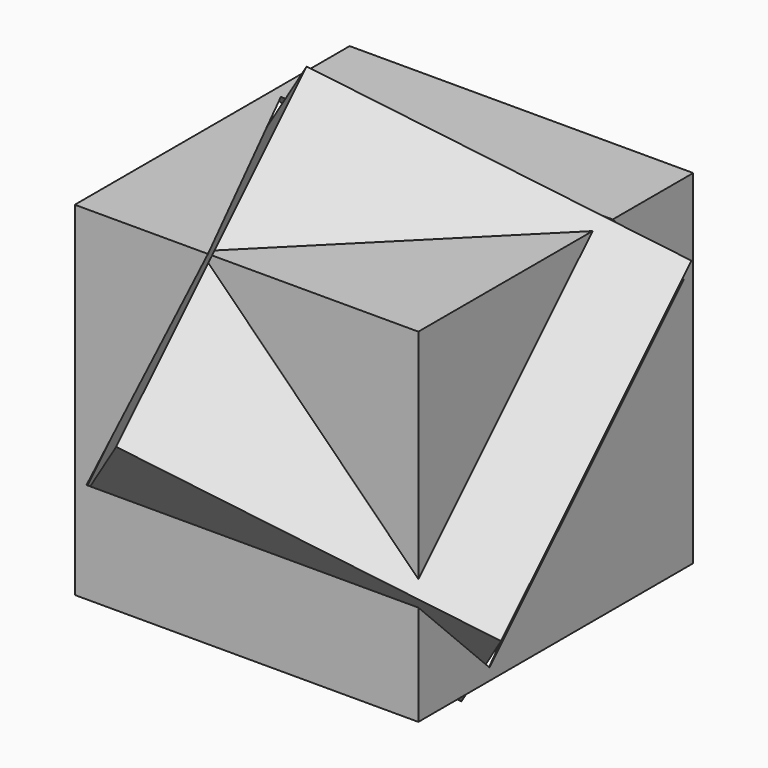
from build123d import *

# Parameters (mm, degrees)
F1_W          = 50
F1_H          = 50
F2_DEPTH      = 25
F5_DEPTH      = 43.3022701892
F5_DEPTH_BACK = 43.3022701892
F6_DEPTH      = 25


with BuildPart() as f2:
    # F1 (on Top) → F2 (new body, symmetric)
    with BuildSketch(Plane.XY):
        Rectangle(F1_W, F1_H)
    extrude(amount=F2_DEPTH, both=True)

    # F4 (on mid) → F5 (cut, two sides)
    with BuildSketch(Plane(origin=(0, 0, 0), x_dir=(-0.8164965809, -0.4082482905, 0.4082482905), z_dir=(-0.5773502692, 0.5773502692, -0.5773502692))) as f5_sk:
        Polygon((-25, -25), (-14.4337567297, -25), (-14.1450815951, -24.5), (-24.5, -24.5), (-24.5, 24.5), (-14.1450815951, 24.5), (-14.4337567297, 25), (-25, 25), align=None)
        Polygon((-14.1450815951, -24.5), (-14.4337567297, -25), (25, -25), (25, 0), (24.5, 0), (24.5, -24.5), align=None)
        Polygon((25, 25), (-14.4337567297, 25), (-14.1450815951, 24.5), (24.5, 24.5), (24.5, 0), (25, 0), align=None)
    extrude(amount=-F5_DEPTH, mode=Mode.SUBTRACT)
    extrude(f5_sk.sketch, amount=F5_DEPTH_BACK, mode=Mode.SUBTRACT)


with BuildPart() as f6:
    # F4 (on mid) → F6 (new body, symmetric)
    with BuildSketch(Plane(origin=(0, 0, 0), x_dir=(-0.8164965809, -0.4082482905, 0.4082482905), z_dir=(-0.5773502692, 0.5773502692, -0.5773502692))):
        Polygon((-14.1450815951, 24.5), (0, 0), (24.5, 0), (24.5, 24.5), align=None)
        Polygon((0, 0), (-14.1450815951, -24.5), (24.5, -24.5), (24.5, 0), align=None)
        Polygon((-24.5, -24.5), (-14.1450815951, -24.5), (0, 0), (-14.1450815951, 24.5), (-24.5, 24.5), align=None)
    extrude(amount=F6_DEPTH, both=True)


solid = Compound([f2.part, f6.part])
